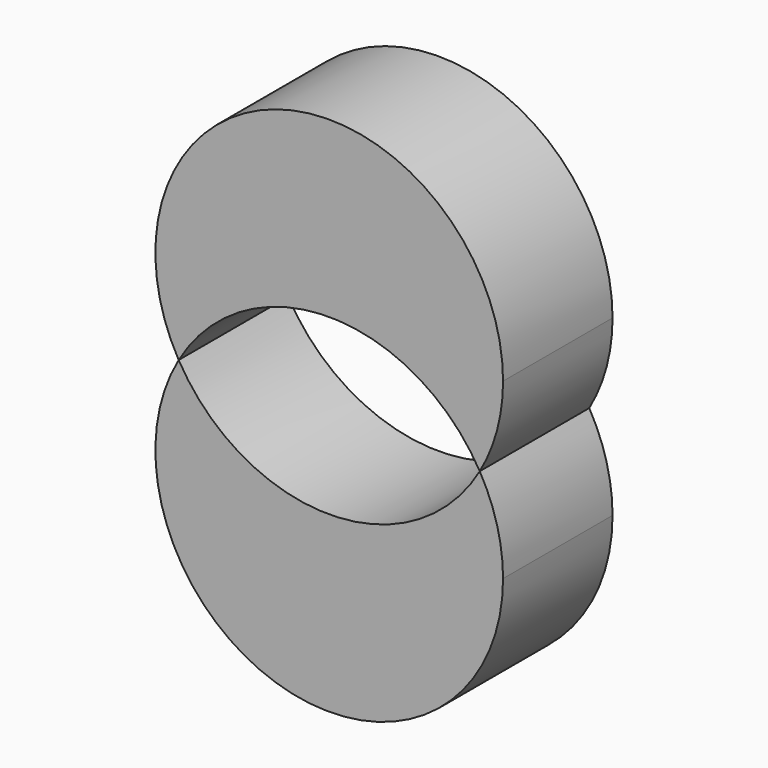
from build123d import *

# Parameters (mm, degrees)
F1_DEPTH = 5


with BuildPart() as f1:
    # F0 (on Front) → F1 (new body, symmetric)
    with BuildSketch(Plane.XZ):
        with BuildLine():
            ThreePointArc((-10.9985226281, 0), (-3.2870018728, -18.6172579939), (12.7, -6.35))
            ThreePointArc((12.7, -6.35), (12.2672579939, -3.0629981272), (10.9985226281, 0))
            ThreePointArc((10.9985226281, 0), (0, -6.35), (-10.9985226281, 0))
        make_face()
    extrude(amount=F1_DEPTH, both=True)


with BuildPart() as f1b:
    # F0 (on Front) → F1, piece 2 (new body, symmetric)
    with BuildSketch(Plane.XZ):
        with BuildLine():
            ThreePointArc((-10.9985226281, 0), (0, 6.35), (10.9985226281, 0))
            ThreePointArc((10.9985226281, 0), (12.2672579939, 3.0629981272), (12.7, 6.35))
            ThreePointArc((12.7, 6.35), (-3.2870018728, 18.6172579939), (-10.9985226281, 0))
        make_face()
    extrude(amount=F1_DEPTH, both=True)


solid = Compound([f1.part, f1b.part])
